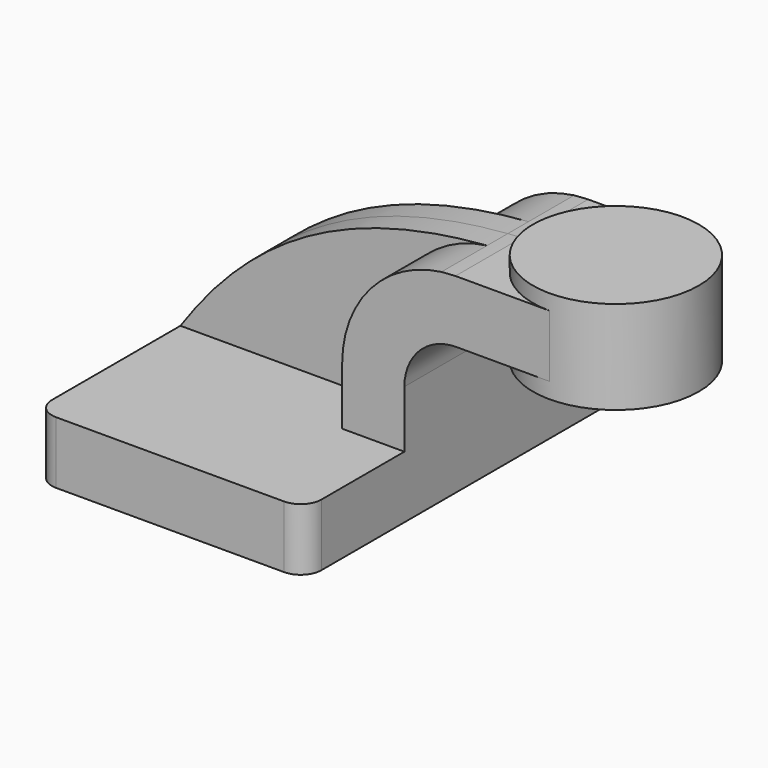
from build123d import *

# Parameters (mm, degrees)
F1_DEPTH = 63.5
F0_W     = 25.4
F0_H     = 19.05
F2_DEPTH = 25.4
F3_DEPTH = 7.9375
F5_R     = 6.35


# Not quite as in the source:
# - a feature names something its author has since deleted; it is built from what else it names


with BuildPart() as f1:
    # F0 (on Front) → F1 (new body, symmetric)
    with BuildSketch(Plane.XZ):
        Polygon((22.225, 9.525), (-41.275, 9.525), (-41.275, -9.525), (41.275, -9.525), (41.275, 9.525), align=None)
    extrude(amount=F1_DEPTH, both=True)



with BuildPart() as f2:
    # F0 (on Front) → F2 (new body, symmetric)
    with BuildSketch(Plane.XZ):
        with BuildLine():
            Line((22.225, 27.0517572581), (22.225, 9.525))
            Line((22.225, 9.525), (41.275, 9.525))
            Line((41.275, 9.525), (41.275, 27.0517572581))
            ThreePointArc((41.275, 27.0517572581), (45.8699924784, 38.2221223064), (56.9949439764, 42.926))
            Line((56.9949439764, 42.926), (60.325, 42.926))
            Line((60.325, 42.926), (60.325, 61.976))
            Line((60.325, 61.976), (56.9200132545, 61.976))
            add(Edge.make_bspline(
                [(52.6300958014, 61.6830450054), (54.0440250085, 61.794890112), (55.4739013545, 61.892529432), (56.9200132545, 61.976)],
                knots=[107.8358858106, 107.8358858106, 107.8358858106, 107.8358858106, 111.3255048452, 111.3255048452, 111.3255048452, 111.3255048452], degree=3))
            ThreePointArc((52.6300958014, 61.6830450054), (30.9048739845, 50.0940875532), (22.225, 27.0517572581))
        make_face()
        with Locations((73.025, 52.451)):
            Rectangle(F0_W, F0_H)
    extrude(amount=F2_DEPTH, both=True)


with BuildPart() as f1_1:
    add(f1.part)

    add(f2.part)  # F3 merges F2
    # F0 (on Front) → F3 (join, symmetric)
    with BuildSketch(Plane.XZ):
        with BuildLine():
            add(Edge.make_bspline(
                [(-41.275, 9.525), (-19.5277563413, 41.2050885172), (8.9369857489, 58.2268178266), (52.6300958014, 61.6830450054)],
                knots=[0, 0, 0, 0, 107.8358858106, 107.8358858106, 107.8358858106, 107.8358858106], degree=3))
            Line((-41.275, 9.525), (22.225, 9.525))
            Line((22.225, 9.525), (22.225, 27.0517572581))
            ThreePointArc((22.225, 27.0517572581), (30.9048739845, 50.0940875532), (52.6300958014, 61.6830450054))
        make_face()
    extrude(amount=F3_DEPTH, both=True)

    # F0 (on Front) → F4 (revolve)
    with BuildSketch(Plane.XZ):
        Polygon((85.725, 66.675), (85.725, 61.976), (85.725, 42.926), (85.725, 38.1), (111.125, 38.1), (111.125, 66.675), align=None)
    revolve(axis=Axis((85.725, 0, 52.3875), (0, 0, -1)))

    # F5
    f5_edges = [f1_1.edges().sort_by_distance(p)[0] for p in [
        (-41.275, -63.5, 0),
        (41.275, -63.5, 0),
        (41.275, 63.5, 0),
        (-41.275, 63.5, 0),
    ]]
    fillet(f5_edges, radius=F5_R)


solid = f1_1.part
